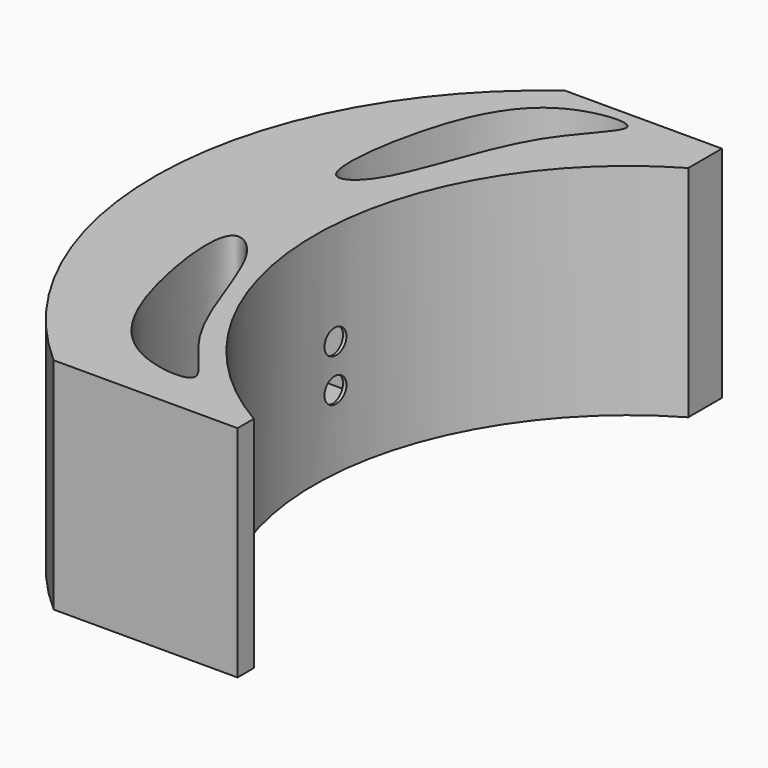
from build123d import *

# Parameters (mm, degrees)
F0_W      = 127
F0_H      = 127
F1_DEPTH  = 44.45
F3_DEPTH  = 44.45
F5_DEPTH  = 44.45
F7_DEPTH  = 46.06675
F8_W      = 32.0189083815
F8_H      = 8.9123969463
F9_DEPTH  = 44.45
F10_W     = 31.75
F10_H     = 19.9242069336
F11_DEPTH = 44.45
F12_W     = 12.7
F12_H     = 25.4
F13_DEPTH = 24.13
F14_R     = 2.54
F14_R_2   = 2.5348059879
F15_DEPTH = 25.4
F17_DEPTH = 44.45
F18_W     = 44.9046668708
F18_H     = 4.3814008621
F19_DEPTH = 44.45
F20_DEPTH = 25


with BuildPart() as f1:
    # F0 (on Top) → F1 (new body)
    with BuildSketch(Plane.XY):
        with Locations((0.2620890737, -5.0497795728)):
            Rectangle(F0_W, F0_H)
    extrude(amount=F1_DEPTH)

    # F2 (on face) → F3 (cut, through all)
    with BuildSketch(Plane.XY.offset(44.45)):
        with BuildLine():
            Line((0.2620890737, 58.4502204272), (-63.2379109263, 58.4502204272))
            Line((-63.2379109263, 58.4502204272), (-63.2379109263, -68.5497795728))
            Line((-63.2379109263, -68.5497795728), (0.2620890737, -68.5497795728))
            ThreePointArc((0.2620890737, -68.5497795728), (-32.0874591554, -5.0497795728), (0.2620890737, 58.4502204272))
        make_face()
    extrude(amount=-F3_DEPTH, mode=Mode.SUBTRACT)

    # F4 (on face) → F5 (cut, through all)
    with BuildSketch(Plane.XY.offset(44.45)):
        with BuildLine():
            Line((63.7620890737, -68.5497795728), (63.7620890737, 58.4502204272))
            ThreePointArc((63.7620890737, 58.4502204272), (0.2620890737, -5.0497795728), (63.7620890737, -68.5497795728))
        make_face()
    extrude(amount=-F5_DEPTH, mode=Mode.SUBTRACT)

    # F6 (on face) → F7 (cut)
    with BuildSketch(Plane.XY.offset(44.45)):
        with BuildLine():
            Line((45.0293794274, -68.5497795728), (45.0293794274, -99.4110107422))
            Line((45.0293794274, -99.4110107422), (83.5961028934, -99.4110107422))
            Line((83.5961028934, -99.4110107422), (83.5961028934, 124.6481090784))
            Line((83.5961028934, 124.6481090784), (45.0293794274, 124.6481090784))
            Line((45.0293794274, 124.6481090784), (45.0293794274, 58.4502204272))
            Line((45.0293794274, 58.4502204272), (63.7620890737, 58.4502204272))
            ThreePointArc((63.7620890737, 58.4502204272), (54.2897526998, 57.7397485638), (45.0293794274, 55.6242312498))
            Line((45.0293794274, 55.6242312498), (45.0293794274, -65.7237903955))
            ThreePointArc((45.0293794274, -65.7237903955), (54.2897526998, -67.8393077095), (63.7620890737, -68.5497795728))
            Line((63.7620890737, -68.5497795728), (45.0293794274, -68.5497795728))
        make_face()
    extrude(amount=-F7_DEPTH, mode=Mode.SUBTRACT)

    # F8 (on face) → F9 (cut, through all)
    with BuildSketch(Plane.XY.offset(44.45)):
        with Locations((48.0215432644, -64.0935810997)):
            Rectangle(F8_W, F8_H)
    extrude(amount=-F9_DEPTH, mode=Mode.SUBTRACT)

    # F10 (on face) → F11 (cut, through all)
    with BuildSketch(Plane.XY.offset(44.45)):
        with Locations((47.8870890737, 48.4881169604)):
            Rectangle(F10_W, F10_H)
    extrude(amount=-F11_DEPTH, mode=Mode.SUBTRACT)

    # F12 (on Right) → F13 (cut)
    with BuildSketch(Plane.YZ):
        with Locations((1.8587405793, 22.86)):
            Rectangle(F12_W, F12_H)
    extrude(amount=-F13_DEPTH, mode=Mode.SUBTRACT)

    # F14 (on face) → F15 (cut)
    with BuildSketch(Plane(origin=(0, 0, 0), x_dir=(0, -1, 0), z_dir=(-1, 0, 0))):
        with Locations((0, 14.9015395448)):
            Circle(F14_R)
        with Locations((0, 23.5572663476)):
            Circle(F14_R_2)
    extrude(amount=-F15_DEPTH, mode=Mode.SUBTRACT)

    # F16 (on face) → F17 (cut, through all)
    with BuildSketch(Plane(origin=(0, 0, 0), x_dir=(1, 0, 0), z_dir=(0, 0, -1))):
        with BuildLine():
            add(Edge.make_bspline(
                [(15.6220020726, -55.0599656999), (14.6747045844, -56.5767938839), (-0.3158932357, -55.1873853804), (-9.8195458276, -35.317884945), (-12.6677317866, -9.6008985203), (-1.3687691608, -16.5812854446), (3.9463942773, -43.3135324972), (16.6526734024, -53.4096379614), (15.6220020726, -55.0599656999)],
                knots=[0, 0, 0, 0, 0.1409804606, 0.3405748592, 0.522571634, 0.6247340088, 0.8466115232, 1, 1, 1, 1], degree=3))
        make_face()
        with BuildLine():
            add(Edge.make_bspline(
                [(15.6220020726, 55.0599656999), (14.6747045844, 56.5767938839), (-0.3158932357, 55.1873853804), (-9.8195458276, 35.317884945), (-12.6677317866, 9.6008985203), (-1.3687691608, 16.5812854446), (3.9463942773, 43.3135324972), (16.6526734024, 53.4096379614), (15.6220020726, 55.0599656999)],
                knots=[0, 0, 0, 0, 0.1409804606, 0.3405748592, 0.522571634, 0.6247340088, 0.8466115232, 1, 1, 1, 1], degree=3))
        make_face()
    extrude(amount=-F17_DEPTH, mode=Mode.SUBTRACT)

    # F18 (on face) → F19 (cut, through all)
    with BuildSketch(Plane.XY.offset(44.45)):
        with Locations((9.5597556382, -66.3590791418)):
            Rectangle(F18_W, F18_H)
    extrude(amount=-F19_DEPTH, mode=Mode.SUBTRACT)

    # F2 (on face) → F20 (cut)
    with BuildSketch(Plane.XY.offset(44.45)):
        with BuildLine():
            Line((0.2620890737, 58.4502204272), (-63.2379109263, 58.4502204272))
            Line((-63.2379109263, 58.4502204272), (-63.2379109263, -68.5497795728))
            Line((-63.2379109263, -68.5497795728), (0.2620890737, -68.5497795728))
            ThreePointArc((0.2620890737, -68.5497795728), (-32.0874591554, -5.0497795728), (0.2620890737, 58.4502204272))
        make_face()
    extrude(amount=-F20_DEPTH, mode=Mode.SUBTRACT)


solid = f1.part
